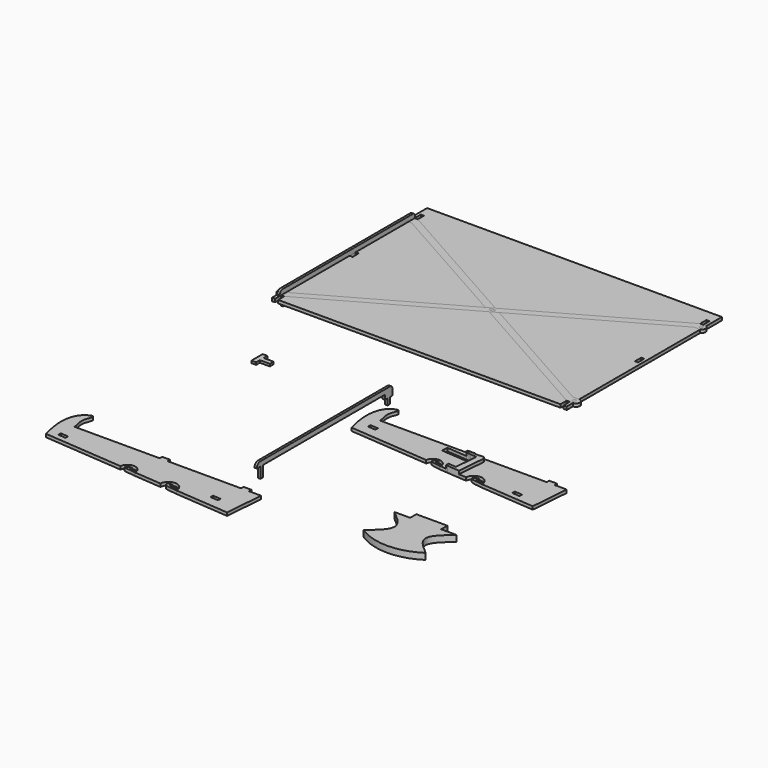
from build123d import *

# Parameters (mm, degrees)
F0_W      = 4
F0_H      = 85
F0_H_2    = 100
F0_H_3    = 15
F0_W_2    = 6
F0_H_4    = 3
F0_W_3    = 3
F0_H_5    = 4
F0_H_6    = 10
F1_DEPTH  = 4
F2_DEPTH  = 4
F3_DEPTH  = 4
F4_DEPTH  = 4
F5_DEPTH  = 4
F6_W      = 4
F6_H      = 2
F6_H_2    = 8
F7_DEPTH  = 3
F0_W_4    = 13
F0_H_7    = 6
F8_DEPTH  = 3
F9_DEPTH  = 8
F0_W_5    = 40
F10_DEPTH = 8


# Not quite as in the source:
# - a feature names something its author has since deleted; it is built from what else it names


with BuildPart() as f1:
    # F0 (on Top) → F1 (new body)
    with BuildSketch(Plane.XY):
        with Locations((184, 47.5)):
            Rectangle(F0_W, F0_H)
        Polygon((182, -115), (182, -105), (8.8780487805, -7.5), (0, -12.5), align=None)
        Polygon((182, 110), (182, 125), (-182, 125), (-182, 110), (-182, 100), (0, -2.5), (182, 100), align=None)
        Polygon((-186, 110), (-186, 125), (-190, 125), (-190, 99.7567328215), (-186, 100), align=None)
        Polygon((182, 90), (182, 100), (0, -2.5), (8.8780487805, -7.5), align=None)
        with Locations((184, -55)):
            Rectangle(F0_W, F0_H_2)
        with Locations((-184, 47.5)):
            Rectangle(F0_W, F0_H)
        with Locations((184, 117.5)):
            Rectangle(F0_W, F0_H_3)
        Polygon((182, 5), (182, 90), (8.8780487805, -7.5), (182, -105), (182, -5), align=None)
        with Locations((-184, -55)):
            Rectangle(F0_W, F0_H_2)
        with Locations((-184, 117.5)):
            Rectangle(F0_W, F0_H_3)
        Polygon((-182, -105), (-8.8780487805, -7.5), (-182, 90), (-182, 5), (-182, -5), align=None)
        Polygon((182, -125), (182, -115), (0, -12.5), (-182, -115), (-182, -125), align=None)
        Polygon((0, -12.5), (-8.8780487805, -7.5), (-182, -105), (-182, -115), align=None)
        Polygon((8.8780487805, -7.5), (0, -2.5), (-8.8780487805, -7.5), (0, -12.5), align=None)
        with Locations((0, -7.5)):
            Rectangle(F0_W_2, F0_H_4, mode=Mode.SUBTRACT)
        Polygon((190, -105), (190, 89.9280673265), (186, 90), (186, 5), (186, -5), (186, -105), align=None)
        Polygon((190, 99.7567328215), (190, 125), (186, 125), (186, 110), (186, 100), align=None)
        Polygon((-182, -115), (-182, -105), (-186, -105), (-190, -105), (-190, -108), (-190, -110), (-190, -112), (-190, -115), (-186, -115), align=None)
        with Locations((-187.6002953053, -110)):
            Rectangle(F0_W_3, F0_H_5, mode=Mode.SUBTRACT)
        Polygon((186, 96.842400074), (186, 100), (182, 100), (182, 90), (186, 90), (186, 92.842400074), align=None)
        with Locations((-188, -120)):
            Rectangle(F0_W, F0_H_6)
        Polygon((190, 89.9280673265), (190, 99.7567328215), (186, 100), (186, 96.842400074), (189, 96.842400074), (189, 92.842400074), (186, 92.842400074), (186, 90), align=None)
        Polygon((190, -108), (190, -105), (186, -105), (186, -115), (190, -115), (190, -112), (190, -110), align=None)
        with Locations((187.6002953053, -110)):
            Rectangle(F0_W_3, F0_H_5, mode=Mode.SUBTRACT)
        with Locations((184, -110)):
            Rectangle(F0_W, F0_H_6)
        with Locations((188, -120)):
            Rectangle(F0_W, F0_H_6)
        Polygon((-8.8780487805, -7.5), (0, -2.5), (-182, 100), (-186, 100), (-190, 99.7567328215), (-190, 89.9280673265), (-186, 90), (-182, 90), align=None)
        with Locations((-187.5, 94.842400074)):
            Rectangle(F0_W_3, F0_H_5, mode=Mode.SUBTRACT)
        Polygon((-186, 90), (-190, 89.9280673265), (-190, -105), (-186, -105), (-186, -5), (-186, 5), align=None)
        with Locations((-187.5, 94.842400074)):
            Rectangle(F0_W_3, F0_H_5)
        with Locations((187.5, 94.842400074)):
            Rectangle(F0_W_3, F0_H_5)
        with Locations((0, -7.5)):
            Rectangle(F0_W_2, F0_H_4)
        with Locations((-187.6002953053, -110)):
            Rectangle(F0_W_3, F0_H_5)
        with Locations((187.6002953053, -110)):
            Rectangle(F0_W_3, F0_H_5)
    extrude(amount=F1_DEPTH)


with BuildPart() as f2:
    # F0 (on Top) → F2 (new body)
    with BuildSketch(Plane.XY):
        Polygon((-8.8780487805, -7.5), (0, -2.5), (-182, 100), (-186, 100), (-190, 99.7567328215), (-190, 89.9280673265), (-186, 90), (-182, 90), align=None)
        with Locations((-187.5, 94.842400074)):
            Rectangle(F0_W_3, F0_H_5, mode=Mode.SUBTRACT)
        with BuildLine():
            Line((-190, 89.9280673265), (-190, 99.7567328215))
            ThreePointArc((-190, 99.7567328215), (-193.0136799284, 94.842400074), (-190, 89.9280673265))
        make_face()
        Polygon((8.8780487805, -7.5), (0, -2.5), (-8.8780487805, -7.5), (0, -12.5), align=None)
        with Locations((0, -7.5)):
            Rectangle(F0_W_2, F0_H_4, mode=Mode.SUBTRACT)
        Polygon((182, -115), (182, -105), (8.8780487805, -7.5), (0, -12.5), align=None)
        with Locations((184, -110)):
            Rectangle(F0_W, F0_H_6)
        with BuildLine():
            ThreePointArc((190, -115), (195, -110), (190, -105))
            Line((190, -105), (190, -108))
            Line((190, -108), (190, -110))
            Line((190, -110), (190, -112))
            Line((190, -112), (190, -115))
        make_face()
        Polygon((190, -108), (190, -105), (186, -105), (186, -115), (190, -115), (190, -112), (190, -110), align=None)
        with Locations((187.6002953053, -110)):
            Rectangle(F0_W_3, F0_H_5, mode=Mode.SUBTRACT)
    extrude(amount=F2_DEPTH)


with BuildPart() as f3:
    # F0 (on Top) → F3 (new body)
    with BuildSketch(Plane.XY):
        Polygon((0, -12.5), (-8.8780487805, -7.5), (-182, -105), (-182, -115), align=None)
        Polygon((-182, -115), (-182, -105), (-186, -105), (-190, -105), (-190, -108), (-190, -110), (-190, -112), (-190, -115), (-186, -115), align=None)
        with Locations((-187.6002953053, -110)):
            Rectangle(F0_W_3, F0_H_5, mode=Mode.SUBTRACT)
        with BuildLine():
            Line((-190, -108), (-190, -105))
            ThreePointArc((-190, -105), (-195, -110), (-190, -115))
            Line((-190, -115), (-190, -112))
            Line((-190, -112), (-190, -110))
            Line((-190, -110), (-190, -108))
        make_face()
        Polygon((8.8780487805, -7.5), (0, -2.5), (-8.8780487805, -7.5), (0, -12.5), align=None)
        with Locations((0, -7.5)):
            Rectangle(F0_W_2, F0_H_4, mode=Mode.SUBTRACT)
        Polygon((182, 90), (182, 100), (0, -2.5), (8.8780487805, -7.5), align=None)
        Polygon((186, 96.842400074), (186, 100), (182, 100), (182, 90), (186, 90), (186, 92.842400074), align=None)
        Polygon((190, 89.9280673265), (190, 99.7567328215), (186, 100), (186, 96.842400074), (189, 96.842400074), (189, 92.842400074), (186, 92.842400074), (186, 90), align=None)
        with BuildLine():
            ThreePointArc((190, 89.9280673265), (193.0136799284, 94.842400074), (190, 99.7567328215))
            Line((190, 99.7567328215), (190, 89.9280673265))
        make_face()
    extrude(amount=F3_DEPTH)


with BuildPart() as f4:
    # F0 (on Top) → F4 (new body)
    with BuildSketch(Plane.XY):
        with BuildLine():
            add(Edge.make_bspline(
                [(49.8015686716, -296.1478759303), (46.8589968738, -286.4347780497), (42.6207177704, -266.6050817405), (48.1286310557, -241.6659618224), (64.8459952885, -234.686504917), (61.9255782339, -244.3155824954), (58.3462310443, -251.0814244627), (62.1620755637, -262.2434173636)],
                knots=[0, 0, 0, 0, 0.2683938838, 0.5089884147, 0.6750731595, 0.7835842714, 1, 1, 1, 1], degree=3))
            Line((49.8015686716, -296.1478759303), (152.3211084378, -304.3494300307))
            ThreePointArc((152.3211084378, -304.3494300307), (161.8149889494, -295.9464355309), (171.9179830594, -303.6063045733))
            add(Edge.make_bspline(
                [(170.4191348813, -305.7972705432), (167.5084843697, -305.459100402), (162.0209498669, -304.50615846), (156.6242420121, -302.8834273201), (159.264314684, -298.9689472068), (164.7928643474, -297.5384906565), (160.1301765875, -303.1739871081), (168.2978812291, -303.1820640304), (171.9179830594, -303.6063045733)],
                knots=[0.0381809149, 0.0381809149, 0.0381809149, 0.0381809149, 0.2301601052, 0.3814132742, 0.5165967893, 0.6514125064, 0.7757871015, 0.99438054, 0.99438054, 0.99438054, 0.99438054], degree=3))
            Line((170.4191348813, -305.7972705432), (179.5617948716, -306.5286825326))
            Line((179.5617948716, -306.5286825326), (179.8807754098, -302.5414213903))
            Line((179.8807754098, -302.5414213903), (181.8595131698, -302.6997202359))
            Line((181.8595131698, -302.6997202359), (189.8340354542, -303.3376813123))
            Line((189.8340354542, -303.3376813123), (191.5884284143, -281.4077450301))
            Line((191.5884284143, -281.4077450301), (151.7158169921, -278.2179396481))
            Line((151.7158169921, -278.2179396481), (152.3537780685, -270.2434173636))
            Line((152.3537780685, -270.2434173636), (178.5988660791, -272.3430220798))
            add(Edge.make_bspline(
                [(180.5835852334, -268.4890198793), (178.4098580205, -269.5477869885), (178.4070418401, -271.1190455608), (178.5988660791, -272.3430220798)],
                knots=[0, 0, 0, 0, 4.3350251536, 4.3350251536, 4.3350251536, 4.3350251536], degree=3))
            Line((180.5835852334, -268.4890198793), (182.5772158045, -268.6485101484))
            Line((182.5772158045, -268.6485101484), (184.5708477445, -268.808000527))
            Line((184.5708477445, -268.808000527), (186.5644769467, -268.9674906866))
            Line((186.5644769467, -268.9674906866), (192.5453700289, -269.4459616034))
            add(Edge.make_bspline(
                [(192.5453700289, -269.4459616034), (195.5556218714, -268.4288090791), (200.0078559925, -268.6975397257), (200.417073794, -271.8363683057), (200.2519499832, -273.4332055147)],
                knots=[0, 0, 0, 0, 0.5690287639, 1, 1, 1, 1], degree=3))
            Line((200.2519499832, -273.4332055147), (197.4895772004, -307.9629035309))
            Line((197.4895772004, -307.9629035309), (207.1316964837, -308.7342722195))
            ThreePointArc((207.1316964837, -308.7342722195), (217.5283200355, -299.0341357305), (228.806867858, -307.6930495306))
            add(Edge.make_bspline(
                [(229.0462508992, -310.4874346316), (225.460478151, -310.1626015051), (217.0341119333, -309.1515944227), (211.6475941226, -306.8336306904), (215.3978967063, -303.8092007334), (221.04269122, -301.8332120443), (215.1746826091, -307.1586108769), (224.8728928605, -307.1423965246), (228.806867858, -307.6930495306)],
                knots=[0, 0, 0, 0, 0.2440017798, 0.3814092584, 0.5162371585, 0.6480678695, 0.7645238284, 0.9819759754, 0.9819759754, 0.9819759754, 0.9819759754], degree=3))
            Line((229.0462508992, -310.4874346316), (299.0056659806, -316.0841816414))
            Line((299.0056659806, -316.0841816414), (302.9929227081, -266.2434173636))
            Line((302.9929227081, -266.2434173636), (287.1939227081, -266.2434173636))
            Line((287.1939227081, -266.2434173636), (287.1939227081, -262.2434173636))
            Line((287.1939227081, -262.2434173636), (277.1939227081, -262.2434173636))
            Line((277.1939227081, -262.2434173636), (277.1939227081, -266.2434173636))
            Line((277.1939227081, -266.2434173636), (182.1939227081, -266.2434173636))
            Line((182.1939227081, -266.2434173636), (182.1939227081, -262.2434173636))
            Line((182.1939227081, -262.2434173636), (172.1939227081, -262.2434173636))
            Line((172.1939227081, -262.2434173636), (172.1939227081, -266.2434173636))
            Line((172.1939227081, -266.2434173636), (62.1620755637, -266.2434173636))
            Line((62.1620755637, -266.2434173636), (62.1620755637, -262.2434173636))
        make_face()
        Polygon((60.327937469, -289.9676202769), (60.6469180072, -285.9803591347), (70.6150708628, -286.7778104802), (70.2960903246, -290.7650716224), align=None, mode=Mode.SUBTRACT)
        Polygon((70.7745611319, -284.7841799091), (60.8064082763, -283.9867285636), (61.1253888145, -279.9994674213), (71.0935416701, -280.7969187668), align=None, mode=Mode.SUBTRACT)
        Polygon((274.6434997836, -307.1128462787), (264.6753469281, -306.3153949332), (264.9943274663, -302.328133791), (274.9624803218, -303.1255851365), align=None, mode=Mode.SUBTRACT)
        Polygon((275.4409511291, -297.1446934232), (275.1219705909, -301.1319545654), (265.1538177354, -300.3345032199), (265.4727982736, -296.3472420777), align=None, mode=Mode.SUBTRACT)
        with BuildLine():
            Line((189.8340354542, -303.3376813123), (189.515054916, -307.3249424545))
            Line((189.515054916, -307.3249424545), (197.4895772004, -307.9629035309))
            Line((197.4895772004, -307.9629035309), (200.2519499832, -273.4332055147))
            add(Edge.make_bspline(
                [(192.5453700289, -269.4459616034), (195.5556218714, -268.4288090791), (200.0078559925, -268.6975397257), (200.417073794, -271.8363683057), (200.2519499832, -273.4332055147)],
                knots=[0, 0, 0, 0, 0.5690287639, 1, 1, 1, 1], degree=3))
            Line((192.5453700289, -269.4459616034), (192.2263894907, -273.4332227456))
            Line((192.2263894907, -273.4332227456), (191.5884284143, -281.4077450301))
            Line((191.5884284143, -281.4077450301), (189.8340354542, -303.3376813123))
        make_face()
        Polygon((265.1538177354, -300.3345032199), (275.1219705909, -301.1319545654), (275.4409511291, -297.1446934232), (265.4727982736, -296.3472420777), align=None)
        Polygon((70.6150708628, -286.7778104802), (60.6469180072, -285.9803591347), (60.327937469, -289.9676202769), (70.2960903246, -290.7650716224), align=None)
        with BuildLine():
            add(Edge.make_bspline(
                [(180.5835852334, -268.4890198793), (178.4098580205, -269.5477869885), (178.4070418401, -271.1190455608), (178.5988660791, -272.3430220798)],
                knots=[0, 0, 0, 0, 4.3350251536, 4.3350251536, 4.3350251536, 4.3350251536], degree=3))
            Line((178.5988660791, -272.3430220798), (182.2582352663, -272.6357712906))
            Line((182.2582352663, -272.6357712906), (182.5772158045, -268.6485101484))
            Line((182.5772158045, -268.6485101484), (180.5835852334, -268.4890198793))
        make_face()
        Polygon((182.2582352663, -272.6357712906), (184.2518672063, -272.7952616692), (184.5708477445, -268.808000527), (182.5772158045, -268.6485101484), align=None)
        Polygon((179.8807754098, -302.5414213903), (179.5617948716, -306.5286825326), (181.5405326316, -306.6869813781), (181.8595131698, -302.6997202359), align=None)
    extrude(amount=F4_DEPTH)


with BuildPart() as f5:
    # F0 (on Top) → F5 (new body)
    with BuildSketch(Plane.XY):
        with BuildLine():
            add(Edge.make_bspline(
                [(-182.0076985974, -498.8467277367), (-184.9544251928, -489.1199153375), (-189.2573919774, -468.5715648347), (-183.4877211676, -444.6685760709), (-166.8897424834, -436.5827475694), (-169.8358977748, -447.1547474925), (-173.4371385852, -453.8560312608), (-169.6471917054, -464.94226917)],
                knots=[0, 0, 0, 0, 0.2687728456, 0.5053431878, 0.6718951014, 0.7850530568, 1, 1, 1, 1], degree=3))
            Line((-182.0076985974, -498.8467277367), (-79.5503017545, -507.0433104088))
            ThreePointArc((-79.5503017545, -507.0433104088), (-69.8315962033, -498.1226454246), (-59.7245469689, -506.6007971764))
            add(Edge.make_bspline(
                [(-59.6153445608, -508.6381052185), (-63.9566419773, -508.2448251904), (-77.5214607218, -507.265500571), (-74.4087544371, -504.4482380823), (-72.2629624222, -502.9897753311), (-66.9619303749, -501.6325172887), (-71.1223373552, -506.2549092453), (-63.3862928229, -506.1375421707), (-59.7245469689, -506.6007971764)],
                knots=[0, 0, 0, 0, 0.295413106, 0.3877460564, 0.5238696175, 0.6611033331, 0.7735329157, 1, 1, 1, 1], degree=3))
            Line((-59.6153445608, -508.6381052185), (-24.6153445608, -511.4381021183))
            ThreePointArc((-24.6153445608, -511.4381021183), (-14.3680795367, -501.3387371042), (-2.8929869166, -510.01778449))
            Line((-2.8929869166, -510.01778449), (-8.0243170232, -510.01778449))
            add(Edge.make_bspline(
                [(-2.6854082786, -513.1924950784), (-6.3476473302, -512.860731244), (-15.5707901142, -512.1395081917), (-19.9756576457, -509.6019759163), (-18.5205013162, -505.9229510755), (-11.3157922349, -505.5221920585), (-17.0350018682, -508.8339783758), (-11.3396075617, -509.4564841526), (-8.0243170232, -510.01778449)],
                knots=[0, 0, 0, 0, 0.24920509, 0.3883791592, 0.5068537883, 0.6505665959, 0.7572317236, 0.9076775898, 0.9076775898, 0.9076775898, 0.9076775898], degree=3))
            Line((-2.6854082786, -513.1924950784), (67.1963987116, -518.7830334478))
            Line((67.1963987116, -518.7830334478), (71.1836554391, -468.94226917))
            Line((71.1836554391, -468.94226917), (55.3846554391, -468.94226917))
            Line((55.3846554391, -468.94226917), (55.3846554391, -464.94226917))
            Line((55.3846554391, -464.94226917), (45.3846554391, -464.94226917))
            Line((45.3846554391, -464.94226917), (45.3846554391, -468.94226917))
            Line((45.3846554391, -468.94226917), (-49.6153445609, -468.94226917))
            Line((-49.6153445609, -468.94226917), (-49.6153445609, -464.94226917))
            Line((-49.6153445609, -464.94226917), (-59.6153445609, -464.94226917))
            Line((-59.6153445609, -464.94226917), (-59.6153445609, -468.94226917))
            Line((-59.6153445609, -468.94226917), (-169.6471917054, -468.94226917))
            Line((-169.6471917054, -468.94226917), (-169.6471917054, -464.94226917))
        make_face()
        Polygon((-171.4813298, -492.6664720833), (-171.1623492618, -488.6792109411), (-161.1941964063, -489.4766622866), (-161.5131769445, -493.4639234288), align=None, mode=Mode.SUBTRACT)
        Polygon((-161.0347061372, -487.4830317155), (-171.0028589927, -486.68558037), (-170.6838784545, -482.6983192278), (-160.715725599, -483.4957705733), align=None, mode=Mode.SUBTRACT)
        Polygon((42.8342325146, -509.8116980851), (32.866079659, -509.0142467396), (33.1850601972, -505.0269855974), (43.1532130528, -505.8244369429), align=None, mode=Mode.SUBTRACT)
        Polygon((43.6316838601, -499.8435452296), (43.3127033219, -503.8308063718), (33.3445504663, -503.0333550263), (33.6635310045, -499.0460938841), align=None, mode=Mode.SUBTRACT)
        Polygon((-170.6838784545, -482.6983192278), (-171.0028589927, -486.68558037), (-161.0347061372, -487.4830317155), (-160.715725599, -483.4957705733), align=None)
        Polygon((33.1850601972, -505.0269855974), (32.866079659, -509.0142467396), (42.8342325146, -509.8116980851), (43.1532130528, -505.8244369429), align=None)
    extrude(amount=F5_DEPTH)


with BuildPart() as f7:
    # F6 (on face) → F7 (new body)
    with BuildSketch(Plane(origin=(-186, 0, 0), x_dir=(0, -1, 0), z_dir=(-1, 0, 0))):
        with BuildLine():
            Line((-96.842400074, 0), (-94.842400074, 0))
            Line((-94.842400074, 0), (-92.842400074, 0))
            Line((-92.842400074, 0), (-92.842400074, 2))
            Line((-92.842400074, 2), (-88.842400074, 2))
            Line((-88.842400074, 2), (-88.842400074, 4))
            Line((-88.842400074, 4), (108, 4))
            Line((108, 4), (108, 0))
            Line((108, 0), (108, -10))
            Line((108, -10), (112, -10))
            Line((112, -10), (112, 0))
            Line((112, 0), (112, 4))
            Line((112, 4), (112, 10))
            Line((112, 10), (-92.842400074, 10))
            Line((-92.842400074, 10), (-96.842400074, 10))
            add(Edge.make_bspline(
                [(-96.842400074, 10), (-98.2749015093, 10.1903006434), (-101.2372882962, 8.7365582585), (-100.842400074, 4)],
                knots=[0, 0, 0, 0, 7.2111025509, 7.2111025509, 7.2111025509, 7.2111025509], degree=3))
            Line((-100.842400074, 4), (-100.842400074, 2))
            Line((-100.842400074, 2), (-96.842400074, 2))
            Line((-96.842400074, 2), (-96.842400074, 0))
        make_face()
        Polygon((-92.842400074, 0), (-94.842400074, 0), (-96.842400074, 0), (-96.842400074, -2), (-92.842400074, -2), align=None)
        with Locations((-90.842400074, -1)):
            Rectangle(F6_W, F6_H)
        with Locations((-90.842400074, 1)):
            Rectangle(F6_W, F6_H)
        with Locations((-98.842400074, 1)):
            Rectangle(F6_W, F6_H)
        with Locations((-98.842400074, -1)):
            Rectangle(F6_W, F6_H)
        with Locations((-94.842400074, -6)):
            Rectangle(F6_W, F6_H_2)
        with BuildLine():
            add(Edge.make_bspline(
                [(112, 10), (115.8096417785, 10.0650973618), (117.6412403584, 7.4755931273), (117.6938042045, 4)],
                knots=[0, 0, 0, 0, 8.2716024033, 8.2716024033, 8.2716024033, 8.2716024033], degree=3))
            Line((112, 10), (112, 4))
            Line((112, 4), (117.6938042045, 4))
        make_face()
    extrude(amount=F7_DEPTH)


with BuildPart() as f7b:
    # F6 (on face) → F7, piece 2 (new body)
    with BuildSketch(Plane(origin=(-186, 0, 0), x_dir=(0, -1, 0), z_dir=(-1, 0, 0))):
        with BuildLine():
            Line((-56.2964718269, -170.8015473992), (-60.2964718269, -170.8015473992))
            add(Edge.make_bspline(
                [(-60.2964718269, -170.8015473992), (-61.7289732622, -170.6112467557), (-64.6913600492, -172.0649891406), (-64.2964718269, -176.8015473992)],
                knots=[0, 0, 0, 0, 7.2111025509, 7.2111025509, 7.2111025509, 7.2111025509], degree=3))
            Line((-64.2964718269, -176.8015473992), (-64.2964718269, -178.8015473992))
            Line((-64.2964718269, -178.8015473992), (-64.2964718269, -180.8015473992))
            Line((-64.2964718269, -180.8015473992), (-64.2964718269, -182.8015473992))
            Line((-64.2964718269, -182.8015473992), (-60.2964718269, -182.8015473992))
            Line((-60.2964718269, -182.8015473992), (-60.2964718269, -190.8015473992))
            Line((-60.2964718269, -190.8015473992), (-56.2964718269, -190.8015473992))
            Line((-56.2964718269, -190.8015473992), (-56.2964718269, -182.8015473992))
            Line((-56.2964718269, -182.8015473992), (-52.2964718269, -182.8015473992))
            Line((-52.2964718269, -182.8015473992), (-52.2964718269, -180.8015473992))
            Line((-52.2964718269, -180.8015473992), (-52.2964718269, -178.8015473992))
            Line((-52.2964718269, -178.8015473992), (-52.2964718269, -176.8015473992))
            Line((-52.2964718269, -176.8015473992), (144.5459282471, -176.8015473992))
            Line((144.5459282471, -176.8015473992), (144.5459282471, -180.8015473992))
            Line((144.5459282471, -180.8015473992), (144.5459282471, -190.8015473992))
            Line((144.5459282471, -190.8015473992), (148.5459282471, -190.8015473992))
            Line((148.5459282471, -190.8015473992), (148.5459282471, -180.8015473992))
            Line((148.5459282471, -180.8015473992), (148.5459282471, -176.8015473992))
            Line((148.5459282471, -176.8015473992), (154.2397324515, -176.8015473992))
            add(Edge.make_bspline(
                [(148.5459282471, -170.8015473992), (152.3555700255, -170.7364500374), (154.1871686054, -173.3259542719), (154.2397324515, -176.8015473992)],
                knots=[0, 0, 0, 0, 8.2716024033, 8.2716024033, 8.2716024033, 8.2716024033], degree=3))
            Line((148.5459282471, -170.8015473992), (-56.2964718269, -170.8015473992))
        make_face()
    extrude(amount=F7_DEPTH)


with BuildPart() as f8:
    # F0 (on Top) → F8 (new body)
    with BuildSketch(Plane.XY):
        with Locations((-109.0757653117, -234.4564558268)):
            Rectangle(F0_W_4, F0_H_7)
        Polygon((-115.5757653117, -243.4564558268), (-115.5757653117, -237.4564558268), (-115.5757653117, -231.4564558268), (-115.5757653117, -225.4564558268), (-121.5757653117, -225.4564558268), (-121.5757653117, -231.4564558268), (-121.5757653117, -237.4564558268), (-121.5757653117, -243.4564558268), align=None)
    extrude(amount=F8_DEPTH)


with BuildPart() as f9:
    # F0 (on Top) → F9 (new body)
    with BuildSketch(Plane.XY):
        with BuildLine():
            Line((189.8340354542, -303.3376813123), (189.515054916, -307.3249424545))
            Line((189.515054916, -307.3249424545), (197.4895772004, -307.9629035309))
            Line((197.4895772004, -307.9629035309), (200.2519499832, -273.4332055147))
            add(Edge.make_bspline(
                [(192.5453700289, -269.4459616034), (195.5556218714, -268.4288090791), (200.0078559925, -268.6975397257), (200.417073794, -271.8363683057), (200.2519499832, -273.4332055147)],
                knots=[0, 0, 0, 0, 0.5690287639, 1, 1, 1, 1], degree=3))
            Line((192.5453700289, -269.4459616034), (192.2263894907, -273.4332227456))
            Line((192.2263894907, -273.4332227456), (191.5884284143, -281.4077450301))
            Line((191.5884284143, -281.4077450301), (189.8340354542, -303.3376813123))
        make_face()
        Polygon((181.8595131698, -302.6997202359), (181.5405326316, -306.6869813781), (189.515054916, -307.3249424545), (189.8340354542, -303.3376813123), align=None)
        Polygon((179.8807754098, -302.5414213903), (179.5617948716, -306.5286825326), (181.5405326316, -306.6869813781), (181.8595131698, -302.6997202359), align=None)
        Polygon((184.2518672063, -272.7952616692), (192.2263894907, -273.4332227456), (192.5453700289, -269.4459616034), (186.5644769467, -268.9674906866), (184.5708477445, -268.808000527), align=None)
        Polygon((182.2582352663, -272.6357712906), (184.2518672063, -272.7952616692), (184.5708477445, -268.808000527), (182.5772158045, -268.6485101484), align=None)
        with BuildLine():
            add(Edge.make_bspline(
                [(180.5835852334, -268.4890198793), (178.4098580205, -269.5477869885), (178.4070418401, -271.1190455608), (178.5988660791, -272.3430220798)],
                knots=[0, 0, 0, 0, 4.3350251536, 4.3350251536, 4.3350251536, 4.3350251536], degree=3))
            Line((178.5988660791, -272.3430220798), (182.2582352663, -272.6357712906))
            Line((182.2582352663, -272.6357712906), (182.5772158045, -268.6485101484))
            Line((182.5772158045, -268.6485101484), (180.5835852334, -268.4890198793))
        make_face()
    extrude(amount=F9_DEPTH)


with BuildPart() as f10:
    # F0 (on Top) → F10 (new body)
    with BuildSketch(Plane.XY):
        Polygon((263.195425272, -418.8381135464), (223.195425272, -418.8381135464), (223.195425272, -443.8381135464), (223.195425272, -468.8381135464), (263.195425272, -468.8381135464), (263.195425272, -443.8381135464), align=None)
        with BuildLine():
            Line((271.6792696714, -418.8381135464), (263.195425272, -418.8381135464))
            Line((263.195425272, -418.8381135464), (263.195425272, -443.8381135464))
            add(Edge.make_bspline(
                [(283.195425272, -418.8381135464), (273.195425272, -427.1714468797), (263.195425272, -435.504780213), (263.195425272, -443.8381135464)],
                knots=[0, 0, 0, 0, 0.5, 0.5, 0.5, 0.5], degree=3))
            Line((283.195425272, -418.8381135464), (271.6792696714, -418.8381135464))
        make_face()
        with BuildLine():
            add(Edge.make_bspline(
                [(263.195425272, -443.8381135464), (263.195425272, -452.1714468797), (273.195425272, -460.504780213), (283.195425272, -468.8381135464)],
                knots=[0.5, 0.5, 0.5, 0.5, 1, 1, 1, 1], degree=3))
            Line((263.195425272, -443.8381135464), (263.195425272, -468.8381135464))
            Line((263.195425272, -468.8381135464), (283.195425272, -468.8381135464))
        make_face()
        with BuildLine():
            Line((223.195425272, -468.8381135464), (223.195425272, -443.8381135464))
            add(Edge.make_bspline(
                [(223.195425272, -443.8381135464), (223.195425272, -452.1714468797), (213.195425272, -460.504780213), (203.195425272, -468.8381135464)],
                knots=[0.5, 0.5, 0.5, 0.5, 1, 1, 1, 1], degree=3))
            Line((203.195425272, -468.8381135464), (223.195425272, -468.8381135464))
        make_face()
        with BuildLine():
            Line((263.195425272, -468.8381135464), (223.195425272, -468.8381135464))
            Line((223.195425272, -468.8381135464), (203.195425272, -468.8381135464))
            ThreePointArc((203.195425272, -468.8381135464), (243.195425272, -480.8381135464), (283.195425272, -468.8381135464))
            Line((283.195425272, -468.8381135464), (263.195425272, -468.8381135464))
        make_face()
        with Locations((243.195425272, -413.8381135464)):
            Rectangle(F0_W_5, F0_H_6)
        with BuildLine():
            Line((223.195425272, -443.8381135464), (223.195425272, -418.8381135464))
            Line((223.195425272, -418.8381135464), (203.195425272, -418.8381135464))
            add(Edge.make_bspline(
                [(203.195425272, -418.8381135464), (213.195425272, -427.1714468797), (223.195425272, -435.504780213), (223.195425272, -443.8381135464)],
                knots=[0, 0, 0, 0, 0.5, 0.5, 0.5, 0.5], degree=3))
        make_face()
    extrude(amount=F10_DEPTH)


solid = Compound([f1.part, f2.part, f3.part, f4.part, f5.part, f7.part, f7b.part, f8.part, f9.part, f10.part])
